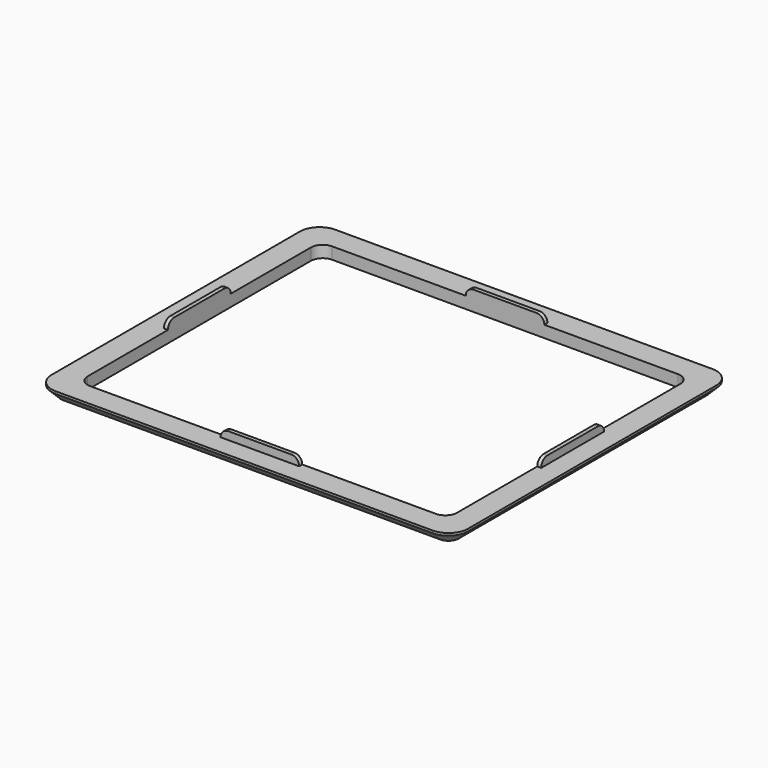
from build123d import *

# Parameters (mm, degrees)
F0_W     = 106
F0_H     = 89
F1_DEPTH = 1
F0_W_2   = 20
F0_H_2   = 1
F0_W_3   = 1
F0_H_3   = 20
F2_DEPTH = 3
F3_DEPTH = 2
F4_R     = 3
F5_R     = 5
F6_SIZE2 = 2.4
F6_SIZE  = 2.4
F7_R     = 1.99999


# Not quite as in the source:
# - a fillet or chamfer is up to 0.001 mm smaller than in the source, because OpenCascade refuses the exact size


with BuildPart() as f1:
    # F0 (on Top) → F1 (new body)
    with BuildSketch(Plane.XY):
        Rectangle(F0_W, F0_H)
        Polygon((-47, 10), (-47, 38.5), (-10, 38.5), (-10, 39.5), (10, 39.5), (10, 38.5), (47, 38.5), (47, 10), (48, 10), (48, -10), (47, -10), (47, -38.5), (10, -38.5), (10, -39.5), (-10, -39.5), (-10, -38.5), (-47, -38.5), (-47, -10), (-48, -10), (-48, 10), align=None, mode=Mode.SUBTRACT)
    extrude(amount=F1_DEPTH)

    # F0 (on Top) → F2 (join)
    with BuildSketch(Plane.XY):
        with Locations((0, 39)):
            Rectangle(F0_W_2, F0_H_2)
        with Locations((-47.5, 0)):
            Rectangle(F0_W_3, F0_H_3)
        with Locations((47.5, 0)):
            Rectangle(F0_W_3, F0_H_3)
        with Locations((0, -39)):
            Rectangle(F0_W_2, F0_H_2)
    extrude(amount=F2_DEPTH)

    # F0 (on Top) → F3 (join)
    with BuildSketch(Plane.XY):
        Rectangle(F0_W, F0_H)
        Polygon((-47, 10), (-47, 38.5), (-10, 38.5), (-10, 39.5), (10, 39.5), (10, 38.5), (47, 38.5), (47, 10), (48, 10), (48, -10), (47, -10), (47, -38.5), (10, -38.5), (10, -39.5), (-10, -39.5), (-10, -38.5), (-47, -38.5), (-47, -10), (-48, -10), (-48, 10), align=None, mode=Mode.SUBTRACT)
        with Locations((0, 39)):
            Rectangle(F0_W_2, F0_H_2)
        with Locations((47.5, 0)):
            Rectangle(F0_W_3, F0_H_3)
        with Locations((-47.5, 0)):
            Rectangle(F0_W_3, F0_H_3)
        with Locations((0, -39)):
            Rectangle(F0_W_2, F0_H_2)
    extrude(amount=-F3_DEPTH)

    # F4
    f4_edges = [f1.edges().sort_by_distance(p)[0] for p in [
        (47, 38.5, -0.5),
        (47, -38.5, -0.5),
        (-47, 38.5, -0.5),
        (-47, -38.5, -0.5),
    ]]
    fillet(f4_edges, radius=F4_R)

    # F5
    f5_edges = [f1.edges().sort_by_distance(p)[0] for p in [
        (-53, -44.5, -0.5),
        (53, -44.5, -0.5),
        (-53, 44.5, -0.5),
        (53, 44.5, -0.5),
    ]]
    fillet(f5_edges, radius=F5_R)

    # F6
    f6_edges = [f1.edges().sort_by_distance(p)[0] for p in [
        (0, -44.5, -2),
    ]]
    chamfer(f6_edges, length=F6_SIZE, length2=F6_SIZE2)

    # F7 (radius 2 in the source; OpenCascade refuses exactly that, so slightly less here)
    f7_edges = [f1.edges().sort_by_distance(p)[0] for p in [
        (10, -39, 3),
        (-10, -39, 3),
        (-47.5, -10, 3),
        (-47.5, 10, 3),
        (-10, 39, 3),
        (10, 39, 3),
        (47.5, 10, 3),
        (47.5, -10, 3),
    ]]
    fillet(f7_edges, radius=F7_R)


solid = f1.part
